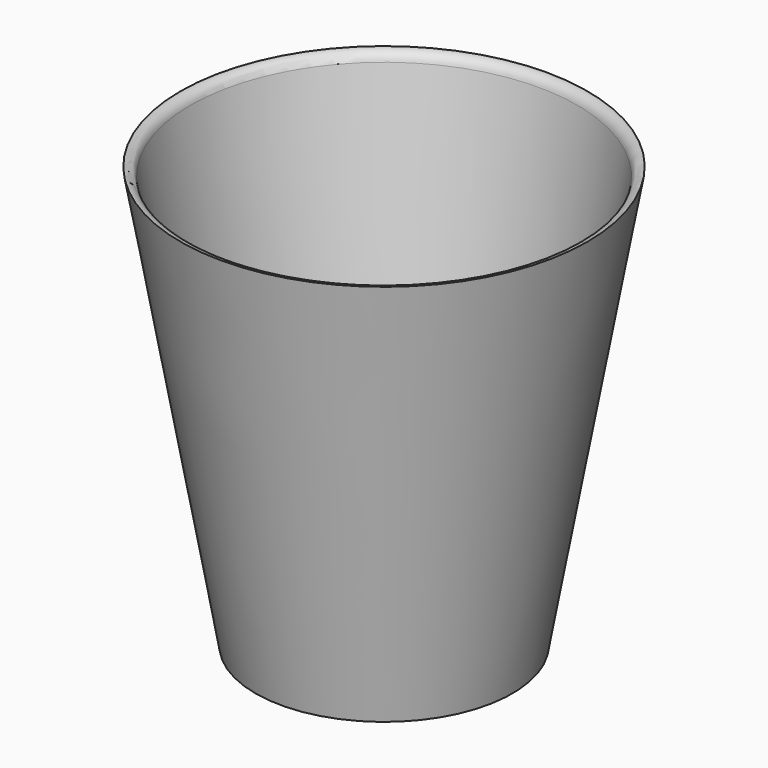
from build123d import *

# Parameters (mm, degrees)
F2_T = -8


# Not quite as in the source:
# - a fillet or chamfer that OpenCascade refuses, or shapes differently, is made with other operations: its cross-section is extruded or revolved along the edge and cut away or added


with BuildPart() as f1:
    # F0 (on Front) → F1 (revolve)
    with BuildSketch(Plane.XZ):
        Polygon((-120, 0), (0, 0), (0, 393.8273733503), (-190, 393.8273733503), align=None)
    revolve(axis=Axis((0, 0, 196.9136866752), (0, 0, -1)))

    # F2
    f2_openings = [f1.faces().sort_by_distance(p)[0] for p in [
        (0, 0, 393.827373),
    ]]
    offset(amount=F2_T, openings=f2_openings)

    # F3: fillet of radius 10 on 1 edges, made by hand

    # F3_s1 → F3_t2 (revolve, cut)
    with BuildSketch(Plane.XZ):
        with BuildLine():
            ThreePointArc((-190, 393.8273733503), (-183.7348569365, 391.4131139305), (-180.408809713, 385.5806122358))
            Line((-180.408809713, 385.5806122358), (-181.8746125421, 393.8273733503))
            Line((-181.8746125421, 393.8273733503), (-190, 393.8273733503))
        make_face()
    revolve(axis=Axis((0, 0, 393.8273733503), (0, 0, -1)), mode=Mode.SUBTRACT)


solid = f1.part
